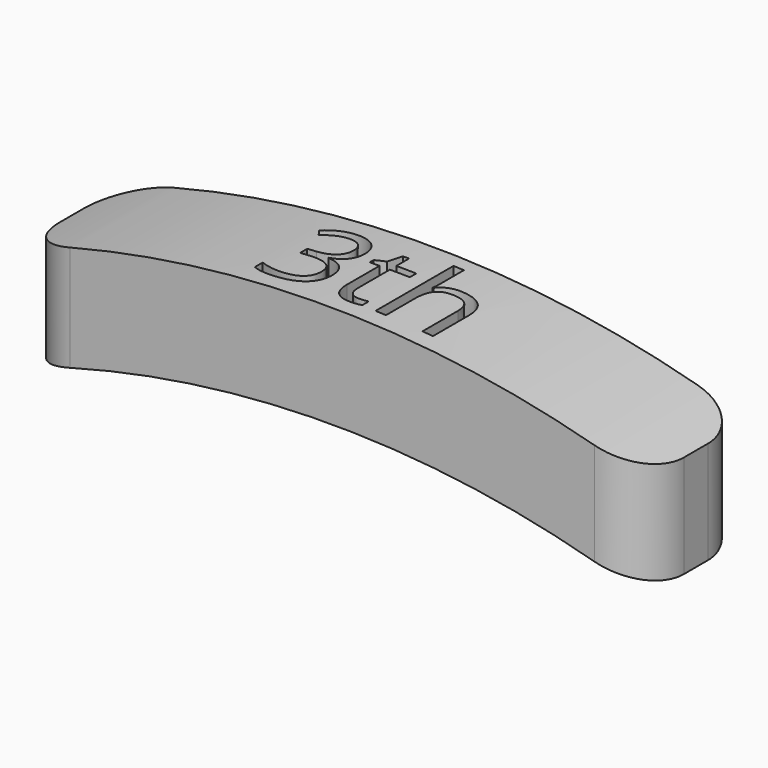
from build123d import *

# Parameters (mm, degrees)
F0_W         = 37.581153214
F0_H         = 7.8032463789
F1_DEPTH     = 9.3
F3_DEPTH     = 36.9
F4_R         = 3
F5_TEXT_SIZE = 7.7235195527
F6_DEPTH     = 31.8
F7_W         = 19.232631661
F7_H         = 3.6202603951
F8_DEPTH     = 7.7


# Not quite as in the source:
# - Text() gives the source's letters only with a copy of the font that has no kerning and outlines rounded to 1/6400 em; it was checked with that copy


with BuildPart() as f1:
    # F0 (on Top) → F1 (new body)
    with BuildSketch(Plane.XY):
        with Locations((18.790576607, -3.9016231894)):
            Rectangle(F0_W, F0_H)
    extrude(amount=F1_DEPTH)

    # F2 (on face) → F3 (intersect)
    with BuildSketch(Plane.XZ.offset(7.8032463789)):
        with BuildLine():
            ThreePointArc((0, 0), (18.790576607, 3.0391537154), (37.581153214, 0))
            Line((37.581153214, 0), (37.581153214, 6.1855874956))
            ThreePointArc((37.581153214, 6.1855874956), (18.8102824914, 9.231635569), (0, 6.4392765053))
            Line((0, 6.4392765053), (0, 0))
        make_face()
    extrude(amount=-F3_DEPTH, mode=Mode.INTERSECT)

    # F4
    f4_edges = [f1.edges().sort_by_distance(p)[0] for p in [
        (37.581153, -7.803246, 3.092794),
        (37.581153, 0, 3.092794),
        (0, 0, 3.219638),
        (0, -7.803246, 3.219638),
    ]]
    fillet(f4_edges, radius=F4_R)

    # F5 (on Top) → F6 (cut)
    with BuildSketch(Plane.XY):
        with Locations((12.7363339998, -6.7269359715)):
            Text('3th', F5_TEXT_SIZE, font='Open Sans', text_align=(TextAlign.LEFT, TextAlign.BOTTOM))
    extrude(amount=F6_DEPTH, mode=Mode.SUBTRACT)

    # F7 (on face) → F8 (join)
    with BuildSketch(Plane(origin=(0, 0, 0), x_dir=(-1, 0, 0), z_dir=(0, 1, 0))):
        with Locations((-18.2977723889, 5.7702451013)):
            Rectangle(F7_W, F7_H)
    extrude(amount=-F8_DEPTH)


solid = f1.part
